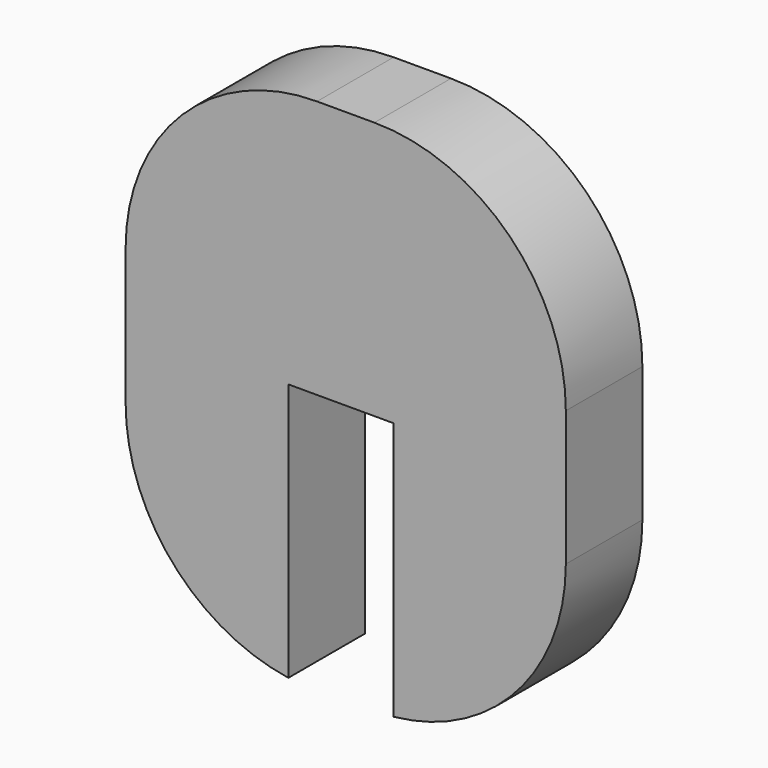
from build123d import *

# Parameters (mm, degrees)
F1_DEPTH    = 5
F2_T1_DEPTH = 55
F2_T3_DEPTH = 54.7482455069
F2_T5_DEPTH = 54.435996907


# Not quite as in the source:
# - a fillet or chamfer that OpenCascade refuses, or shapes differently, is made with other operations: its cross-section is extruded or revolved along the edge and cut away or added


with BuildPart() as f1:
    # F0 (on Front) → F1 (new body)
    with BuildSketch(Plane.XZ):
        Polygon((2.5022388734, -13.5), (11.5, -13.5), (11.5, 13.5), (-11.5, 13.5), (-11.5, -13.5), (-2.9977611266, -13.5), (-2.9977611266, 0), (2.5022388734, 0), align=None)
    extrude(amount=F1_DEPTH)

    # F2: fillet of radius 10 on 4 edges, made by hand

    # F2_s2 → F2_t1 (cut)
    with BuildSketch(Plane.XZ.offset(-25)):
        with BuildLine():
            ThreePointArc((-1.5, 13.5), (-8.5710678119, 10.5710678119), (-11.5, 3.5))
            Line((-11.5, 3.5), (-11.5, 13.5))
            Line((-11.5, 13.5), (-1.5, 13.5))
        make_face()
        with BuildLine():
            ThreePointArc((11.5, 3.5), (8.5710678119, 10.5710678119), (1.5, 13.5))
            Line((1.5, 13.5), (11.5, 13.5))
            Line((11.5, 13.5), (11.5, 3.5))
        make_face()
    extrude(amount=F2_T1_DEPTH, mode=Mode.SUBTRACT)

    # F2_s4 → F2_t3 (cut)
    with BuildSketch(Plane.XZ.offset(-24.8741227535)):
        with BuildLine():
            ThreePointArc((2.5022388734, -13.5), (8.9169531728, -10.2577204004), (11.5, -3.5503508986))
            Line((11.5, -3.5503508986), (11.5, -13.5))
            Line((11.5, -13.5), (2.5022388734, -13.5))
        make_face()
    extrude(amount=F2_T3_DEPTH, mode=Mode.SUBTRACT)

    # F2_s6 → F2_t5 (cut)
    with BuildSketch(Plane.XZ.offset(-24.7179984535)):
        with BuildLine():
            ThreePointArc((-11.5, -3.6128006186), (-9.0821372734, -10.132861536), (-2.9977611266, -13.5))
            Line((-2.9977611266, -13.5), (-11.5, -13.5))
            Line((-11.5, -13.5), (-11.5, -3.6128006186))
        make_face()
    extrude(amount=F2_T5_DEPTH, mode=Mode.SUBTRACT)


solid = f1.part
